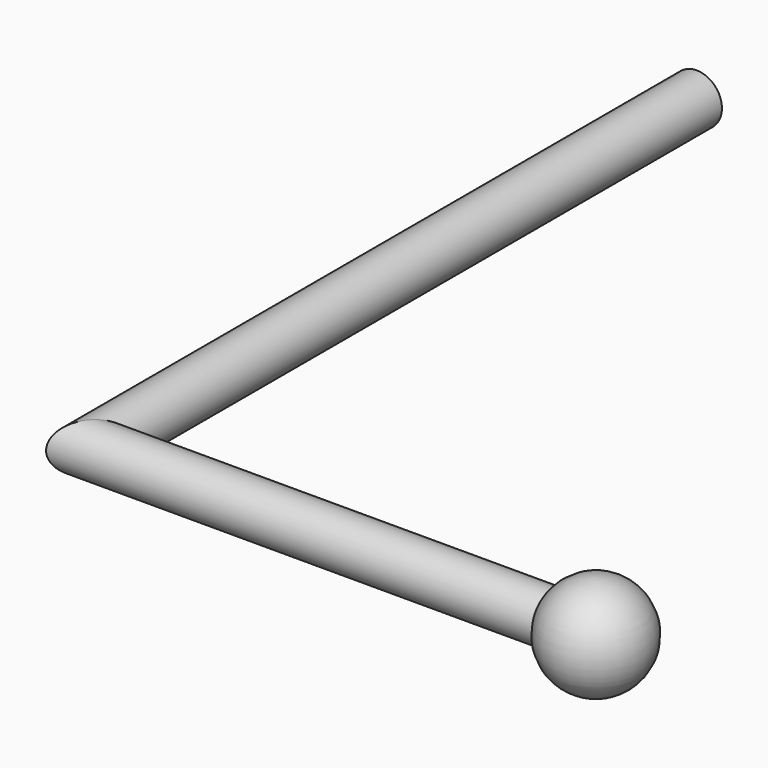
from build123d import *

# Parameters (mm, degrees)
F1_R = 5


# Not quite as in the source:
# - ends of sketch curves that miss each other by under 0.0002 mm in the source are joined


with BuildPart() as f2:
    # F2: sweep along a path in F0
    with BuildLine(Plane.XY) as f2_path:
        Line((0, 0), (0, -150))
        Line((0, -150), (100, -150))
    # F1 (on Front) → F2 (sweep)
    with BuildSketch(Plane.XZ):
        Circle(F1_R)
    sweep(path=f2_path.line, transition=Transition.RIGHT)

    # F3 (on face) → F4 (revolve)
    with BuildSketch(Plane.YZ.offset(100)):
        with BuildLine():
            Line((-150, 10), (-150, 5))
            ThreePointArc((-150, 5), (-146.4644660941, 3.5355339059), (-145, 0))
            ThreePointArc((-145, 0), (-146.4644660941, -3.5355339059), (-150, -5))
            Line((-150, -5), (-150, -10))
            ThreePointArc((-150, -10), (-139.9999966098, 0), (-150, 10))
        make_face()
        with BuildLine():
            Line((-150, 5), (-150, 0))
            Line((-150, 0), (-150, -5))
            ThreePointArc((-150, -5), (-146.4644660941, -3.5355339059), (-145, 0))
            ThreePointArc((-145, 0), (-146.4644660941, 3.5355339059), (-150, 5))
        make_face()
    revolve(axis=Axis((100, -150, 5), (0, 0, 1)))


solid = f2.part
